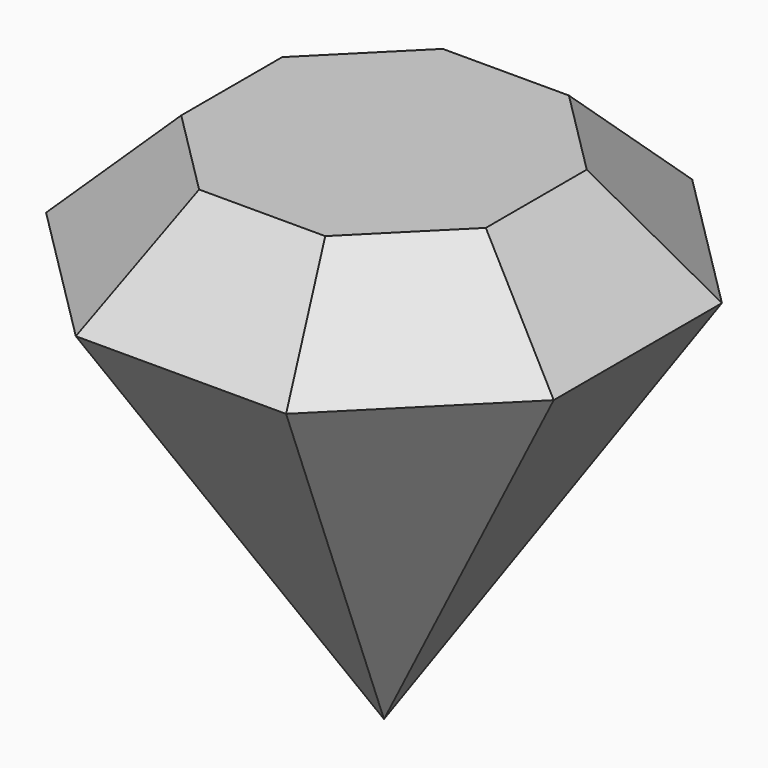
from build123d import *

# Parameters (mm, degrees)
F1_DEPTH = 12.7
F2_SIZE2 = 12.69999
F2_SIZE  = 12.69999


# Not quite as in the source:
# - a fillet or chamfer is up to 0.001 mm smaller than in the source, because OpenCascade refuses the exact size


with BuildPart() as f1:
    # F0 (on Top) → F1 (new body)
    with BuildSketch(Plane.XY):
        Polygon((-31.75, 13.1512806053), (-31.75, -13.1512806053), (-13.1512806053, -31.75), (13.1512806053, -31.75), (31.75, -13.1512806053), (31.75, 13.1512806053), (13.1512806053, 31.75), (-13.1512806053, 31.75), align=None)
    extrude(amount=F1_DEPTH)

    # F2 (size 12.7 and 12.7 in the source; OpenCascade refuses exactly that, so slightly less here)
    f2_edges = [f1.edges().sort_by_distance(p)[0] for p in [
        (-22.45064, 22.45064, 12.7),
        (-31.75, 0, 12.7),
        (-22.45064, -22.45064, 12.7),
        (0, -31.75, 12.7),
        (22.45064, -22.45064, 12.7),
        (31.75, 0, 12.7),
        (22.45064, 22.45064, 12.7),
        (0, 31.75, 12.7),
    ]]
    chamfer(f2_edges, length=F2_SIZE, length2=F2_SIZE2)

    # F1_face (on face) → F5 section 0
    with BuildSketch(Plane(origin=(0, 0, 0), x_dir=(1, 0, 0), z_dir=(0, 0, -1)), mode=Mode.PRIVATE) as f5_s0:
        Polygon((-31.75, -13.1512806053), (-13.1512806053, -31.75), (13.1512806053, -31.75), (31.75, -13.1512806053), (31.75, 13.1512806053), (13.1512806053, 31.75), (-13.1512806053, 31.75), (-31.75, 13.1512806053), align=None)
    loft([f5_s0.sketch, Vertex(0, 0, -50.8)])


solid = f1.part
